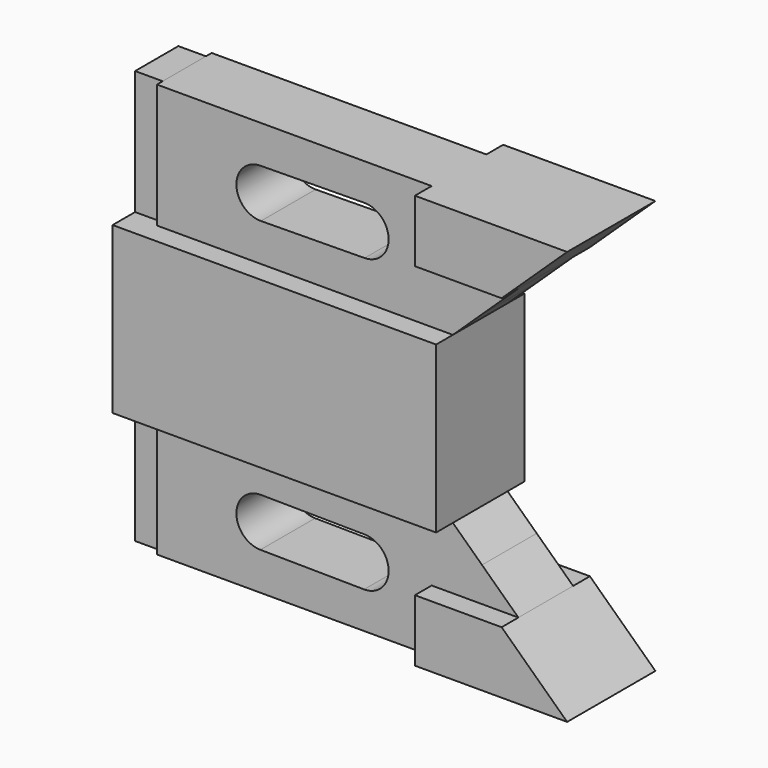
from build123d import *

# Parameters (mm, degrees)
F1_DEPTH = 12.7
F2_DEPTH = 7.874
F0_W     = 6.35
F0_H     = 22.225
F0_H_2   = 6.35
F3_DEPTH = 6.223


with BuildPart() as f1:
    # F0 (on Front) → F1 (new body, symmetric)
    with BuildSketch(Plane.XZ):
        Polygon((62.5320133061, 26.9085878074), (27.4800133061, 26.9085878074), (27.4800133061, 12.6210878074), (47.4474663035, 12.6210878074), align=None)
    extrude(amount=F1_DEPTH, both=True)

    # F0 (on Front) → F2 (join, symmetric)
    with BuildSketch(Plane.XZ):
        Polygon((27.4800133061, 26.9085878074), (-35.7659866939, 26.9085878074), (-35.7659866939, 4.6835878074), (39.0671624131, 4.6835878074), (47.4474663035, 12.6210878074), (27.4800133061, 12.6210878074), align=None)
        with BuildLine():
            ThreePointArc((-11.8286832659, 7.0334240837), (-17.4776504176, 12.5597843794), (-11.9512901219, 18.2087515312))
            Line((-11.9512901219, 18.2087515312), (11.9232730614, 18.4706843599))
            ThreePointArc((11.9232730614, 18.4706843599), (15.9141553755, 16.8559482441), (17.5725764894, 12.8830206361))
            ThreePointArc((17.5725764894, 12.8830206361), (15.9575040974, 8.95344175), (12.0458799174, 7.2953569124))
            Line((12.0458799174, 7.2953569124), (-11.8286832659, 7.0334240837))
        make_face(mode=Mode.SUBTRACT)
        Polygon((39.0671624131, 4.6835878074), (-35.7659866939, 4.6835878074), (-35.7659866939, -1.6664121926), (32.3629193008, -1.6664121926), align=None)
    extrude(amount=F2_DEPTH, both=True)


with BuildPart() as f1b:
    # F0 (on Front) → F1, piece 2 (new body, symmetric)
    with BuildSketch(Plane.XZ):
        Polygon((-35.7659866939, -1.6664121926), (-42.1159866939, -1.6664121926), (-42.1159866939, -20.7164121926), (32.3629193008, -20.7164121926), (32.3629193008, -1.6664121926), align=None)
    extrude(amount=F1_DEPTH, both=True)



with BuildPart() as f3:
    # F0 (on Front) → F3 (new body, symmetric)
    with BuildSketch(Plane.XZ):
        with Locations((-38.9409866939, 15.7960878074)):
            Rectangle(F0_W, F0_H)
        with Locations((-38.9409866939, 1.5085878074)):
            Rectangle(F0_W, F0_H_2)
    extrude(amount=F3_DEPTH, both=True)


with BuildPart() as f1b_1:
    add(f1b.part)
    # F4: F1, F1b, F3 across face
    add(f1.part.mirror(Plane(origin=(-4.8765336965, 0, -20.7164121926), x_dir=(1, 0, 0), z_dir=(0, 0, -1))))
    add(f1b.part.mirror(Plane(origin=(-4.8765336965, 0, -20.7164121926), x_dir=(1, 0, 0), z_dir=(0, 0, -1))))
    add(f3.part.mirror(Plane(origin=(-4.8765336965, 0, -20.7164121926), x_dir=(1, 0, 0), z_dir=(0, 0, -1))))


solid = Compound([f1.part, f3.part, f1b_1.part])
